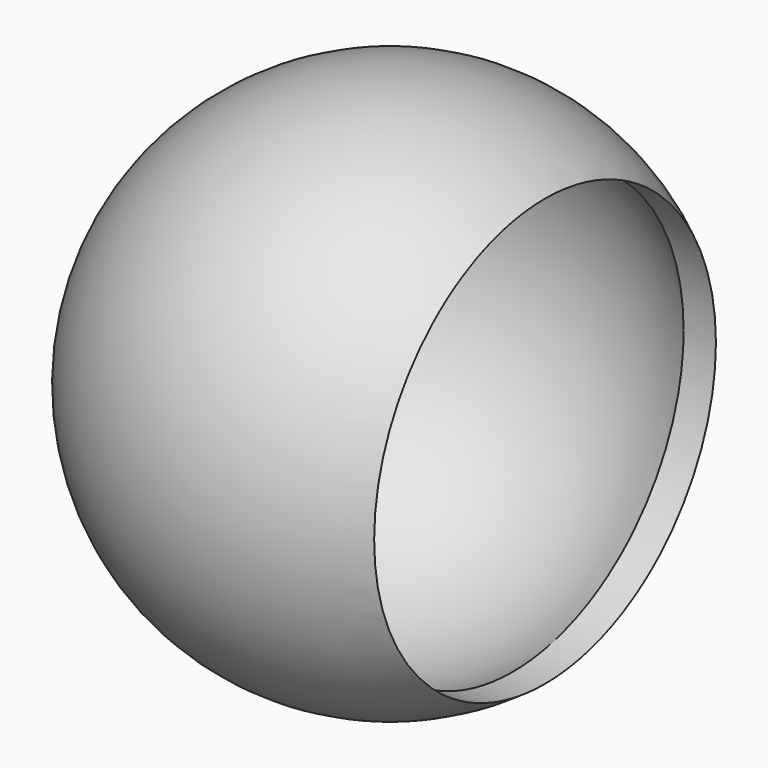
from build123d import *

# Parameters (mm, degrees)
F2_R     = 24.28
F3_DEPTH = 38.8


# Not quite as in the source:
# - a feature names something its author has since deleted; it is built from what else it names


with BuildPart() as f1:
    # F0 (on Front) → F1 (revolve)
    with BuildSketch(Plane.XZ):
        with BuildLine():
            Line((0.1179237399, -27.9997682323), (0.1179237399, -29.9997682323))
            ThreePointArc((0.1179237399, -29.9997682323), (29.999942058, 0.0589619838), (0, 30))
            Line((0, 30), (0, 28))
            ThreePointArc((0, 28), (27.9999461967, 0.0589537232), (0.1179237399, -27.9997682323))
        make_face()
    revolve(axis=Axis((0, 0, 40.6766095488), (0, 0, -1)))

    # F2 (on Right) → F3 (cut)
    with BuildSketch(Plane.YZ):
        Circle(F2_R)
    extrude(amount=F3_DEPTH, mode=Mode.SUBTRACT)


solid = f1.part
